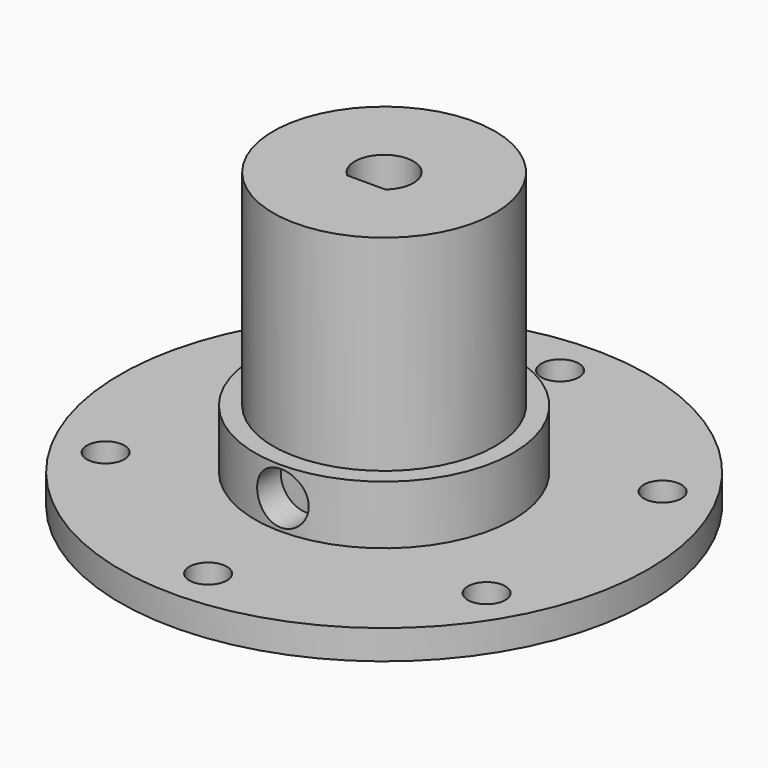
from build123d import *

# Parameters (mm, degrees)
F0_R      = 28.575
F0_R_2    = 2.032
F1_DEPTH  = 3.175
F2_R      = 13.97
F3_DEPTH  = 6.35
F4_R      = 12.0015
F5_DEPTH  = 22.225
F7_DEPTH  = 31.75
F9_R      = 1.4224
F10_DEPTH = 0.3175
F11_R     = 2.794
F12_DEPTH = 3.81


with BuildPart() as f1:
    # F0 (on Top) → F1 (new body)
    with BuildSketch(Plane.XY):
        Circle(F0_R)
        with Locations((-20.6222299276, -11.90625)):
            Circle(F0_R_2, mode=Mode.SUBTRACT)
        with Locations((0, -23.8125)):
            Circle(F0_R_2, mode=Mode.SUBTRACT)
        with Locations((20.6222299276, -11.90625)):
            Circle(F0_R_2, mode=Mode.SUBTRACT)
        with Locations((-20.6222299276, 11.90625)):
            Circle(F0_R_2, mode=Mode.SUBTRACT)
        with Locations((20.6222299276, 11.90625)):
            Circle(F0_R_2, mode=Mode.SUBTRACT)
        with Locations((0, 23.8125)):
            Circle(F0_R_2, mode=Mode.SUBTRACT)
    extrude(amount=F1_DEPTH)

    # F2 (on face) → F3 (join)
    with BuildSketch(Plane.XY.offset(3.175)):
        Circle(F2_R)
    extrude(amount=F3_DEPTH)

    # F4 (on face) → F5 (join)
    with BuildSketch(Plane.XY.offset(9.525)):
        Circle(F4_R)
    extrude(amount=F5_DEPTH)

    # F6 (on face) → F7 (cut, through all)
    with BuildSketch(Plane(origin=(0, 0, 0), x_dir=(1, 0, 0), z_dir=(0, 0, -1))):
        with BuildLine():
            ThreePointArc((-2.0635057548, 2.413), (-1.3283437485, -2.8837697352), (3.175, 0))
            ThreePointArc((3.175, 0), (2.8837697352, 1.3283437485), (2.0635057548, 2.413))
            Line((2.0635057548, 2.413), (0, 2.413))
            Line((0, 2.413), (-2.0635057548, 2.413))
        make_face()
    extrude(amount=-F7_DEPTH, mode=Mode.SUBTRACT)

    # F9 (on offset) → F10 (cut, through all)
    with BuildSketch(Plane.XZ.offset(14.2875)):
        with Locations((0, 6.35)):
            Circle(F9_R)
    extrude(amount=-F10_DEPTH, mode=Mode.SUBTRACT)

    # F11 (on offset) → F12 (cut)
    with BuildSketch(Plane.XZ.offset(14.2875)):
        with Locations((0, 6.35)):
            Circle(F11_R)
    extrude(amount=-F12_DEPTH, mode=Mode.SUBTRACT)


solid = f1.part
